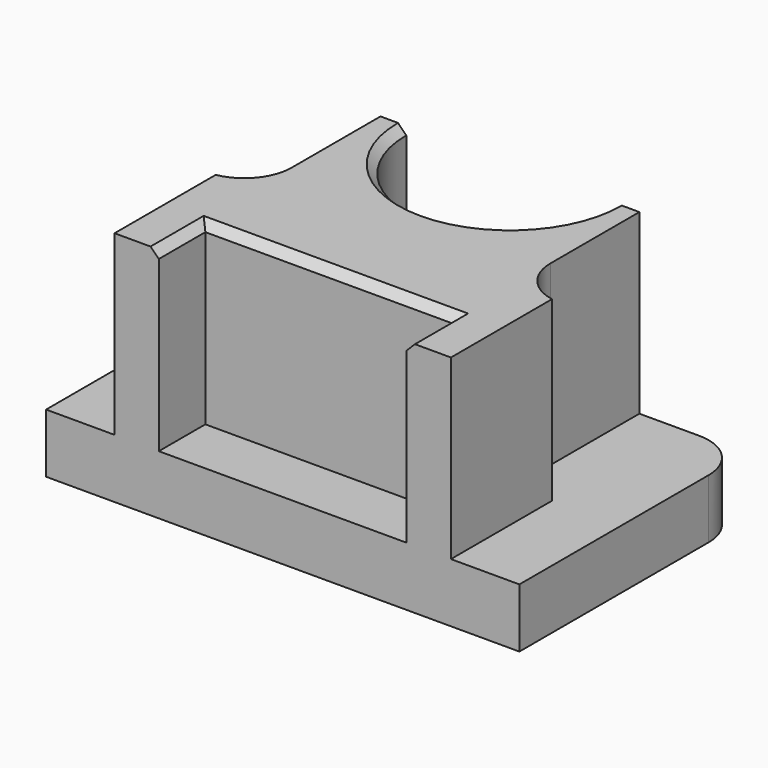
from build123d import *

# Parameters (mm, degrees)
F1_DEPTH     = 19.05
F0_W         = 26.6001702666
F0_H         = 6.2427259982
F2_DEPTH     = 6.35
F3_T1_DEPTH  = 19.05
F3_T6_DEPTH  = 31.5386260012
F3_T8_DEPTH  = 31.75
F3_T10_DEPTH = 31.75
F4_SIZE      = 0.889


# Not quite as in the source:
# - a fillet or chamfer that OpenCascade refuses, or shapes differently, is made with other operations: its cross-section is extruded or revolved along the edge and cut away or added


with BuildPart() as f1:
    # F0 (on Top) → F1 (new body)
    with BuildSketch(Plane.XY):
        with BuildLine():
            Line((7.349026072, 13.5670155287), (7.349026072, 0))
            Line((7.349026072, 0), (12.0999148667, 0))
            Line((12.0999148667, 0), (12.0999148667, 6.2427259982))
            Line((12.0999148667, 6.2427259982), (38.7000851333, 6.2427259982))
            Line((38.7000851333, 6.2427259982), (38.7000851333, 0))
            Line((38.7000851333, 0), (43.450973928, 0))
            Line((43.450973928, 0), (43.450973928, 13.5670155287))
            Line((43.450973928, 13.5670155287), (39.2939448357, 13.5670155287))
            Line((39.2939448357, 13.5670155287), (39.2939448357, 30.48))
            Line((39.2939448357, 30.48), (36.5231766516, 30.48))
            ThreePointArc((36.5231766516, 30.48), (25.4, 19.3568233484), (14.2768233484, 30.48))
            Line((14.2768233484, 30.48), (11.5060551643, 30.48))
            Line((11.5060551643, 30.48), (11.5060551643, 13.5670155287))
            Line((11.5060551643, 13.5670155287), (7.349026072, 13.5670155287))
        make_face()
    extrude(amount=F1_DEPTH)

    # F0 (on Top) → F2 (join)
    with BuildSketch(Plane.XY):
        Polygon((0, 30.48), (0, 0), (7.349026072, 0), (7.349026072, 13.5670155287), (11.5060551643, 13.5670155287), (11.5060551643, 30.48), align=None)
        with Locations((25.4, 3.1213629991)):
            Rectangle(F0_W, F0_H)
        Polygon((43.450973928, 13.5670155287), (43.450973928, 0), (50.8, 0), (50.8, 30.48), (39.2939448357, 30.48), (39.2939448357, 13.5670155287), align=None)
        with BuildLine():
            Line((7.349026072, 13.5670155287), (7.349026072, 0))
            Line((7.349026072, 0), (12.0999148667, 0))
            Line((12.0999148667, 0), (12.0999148667, 6.2427259982))
            Line((12.0999148667, 6.2427259982), (38.7000851333, 6.2427259982))
            Line((38.7000851333, 6.2427259982), (38.7000851333, 0))
            Line((38.7000851333, 0), (43.450973928, 0))
            Line((43.450973928, 0), (43.450973928, 13.5670155287))
            Line((43.450973928, 13.5670155287), (39.2939448357, 13.5670155287))
            Line((39.2939448357, 13.5670155287), (39.2939448357, 30.48))
            Line((39.2939448357, 30.48), (36.5231766516, 30.48))
            ThreePointArc((36.5231766516, 30.48), (25.4, 19.3568233484), (14.2768233484, 30.48))
            Line((14.2768233484, 30.48), (11.5060551643, 30.48))
            Line((11.5060551643, 30.48), (11.5060551643, 13.5670155287))
            Line((11.5060551643, 13.5670155287), (7.349026072, 13.5670155287))
        make_face()
    extrude(amount=-F2_DEPTH)

    # F3: fillet of radius 5.08 on 4 edges, made by hand

    # F3_s2 → F3_t1 (join)
    with BuildSketch(Plane.XY):
        with BuildLine():
            ThreePointArc((7.349026072, 13.5670155287), (10.3308658007, 15.3130269169), (11.5060551643, 18.5624659292))
            Line((11.5060551643, 18.5624659292), (11.5060551643, 13.5670155287))
            Line((11.5060551643, 13.5670155287), (7.349026072, 13.5670155287))
        make_face()
    extrude(amount=F3_T1_DEPTH)


with BuildPart() as f3_tool4:
    # F3_s5 → F3_t6 (new body)
    with BuildSketch(Plane.XY.offset(-12.4886260012)):
        with BuildLine():
            ThreePointArc((43.450973928, 13.5670155287), (40.4691341993, 15.3130269169), (39.2939448357, 18.5624659292))
            Line((39.2939448357, 18.5624659292), (39.2939448357, 13.5670155287))
            Line((39.2939448357, 13.5670155287), (43.450973928, 13.5670155287))
        make_face()
    extrude(amount=F3_T6_DEPTH)

    split(bisect_by=Plane.XY.offset(-6.35), keep=Keep.TOP)


with BuildPart() as f1_1:
    add(f1.part)

    # F3_t3: union F3_tool4
    add(f3_tool4.part)

    # F3_s9 → F3_t8 (cut)
    with BuildSketch(Plane.XY.offset(-19.05)):
        with BuildLine():
            ThreePointArc((5.08, 30.48), (1.4878975516, 28.9921024484), (0, 25.4))
            Line((0, 25.4), (0, 30.48))
            Line((0, 30.48), (5.08, 30.48))
        make_face()
    extrude(amount=F3_T8_DEPTH, mode=Mode.SUBTRACT)

    # F3_s11 → F3_t10 (cut)
    with BuildSketch(Plane.XY.offset(-19.05)):
        with BuildLine():
            ThreePointArc((45.72, 30.48), (49.3121024484, 28.9921024484), (50.8, 25.4))
            Line((50.8, 25.4), (50.8, 30.48))
            Line((50.8, 30.48), (45.72, 30.48))
        make_face()
    extrude(amount=F3_T10_DEPTH, mode=Mode.SUBTRACT)

    # F4
    f4_edges = [f1_1.edges().sort_by_distance(p)[0] for p in [
        (25.4, 19.356823, 19.05),
        (25.4, 6.242726, 19.05),
        (38.700085, 3.121363, 19.05),
        (12.099915, 3.121363, 19.05),
    ]]
    chamfer(f4_edges, length=F4_SIZE)


solid = f1_1.part
